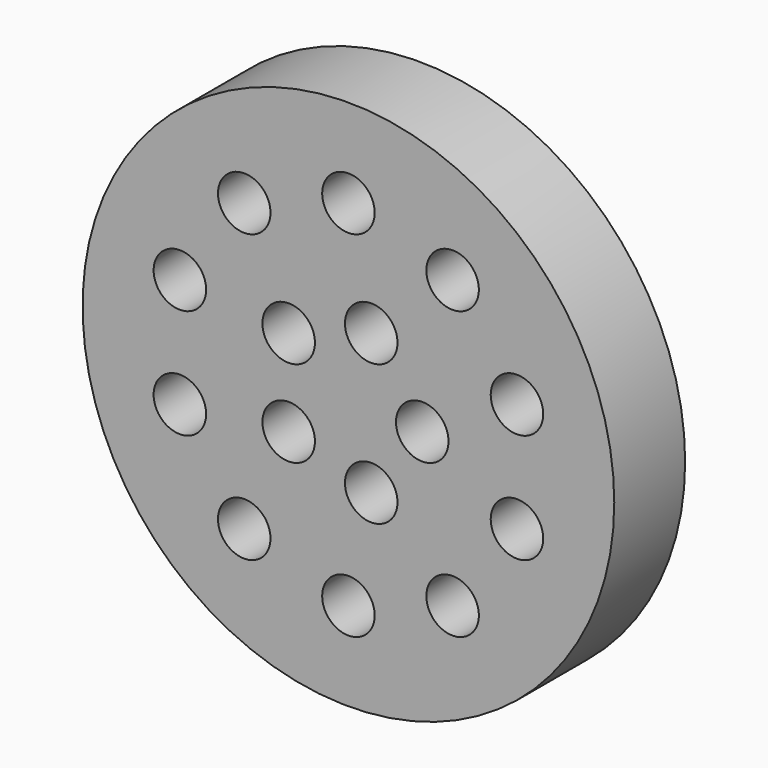
from build123d import *

# Parameters (mm, degrees)
F0_R     = 9
F1_DEPTH = 3
F3_D     = 1.778
F3_DEPTH = 15
F3_TIP   = 0.5341650903


# Not quite as in the source:
# - a feature names something its author has since deleted; it is built from what else it names


with BuildPart() as f1:
    # F0 (on Front) → F1 (new body)
    with BuildSketch(Plane.XZ):
        Circle(F0_R)
    extrude(amount=F1_DEPTH)

    # F3
    with Locations(Plane.XZ.offset(3)):
        with Locations((-3.5267115138, 4.8541019662), (-5.7063390978, 1.8541019662), (-5.7063390978, -1.8541019662), (-3.5267115138, -4.8541019662), (0, -6), (3.5267115138, -4.8541019662), (5.7063390978, -1.8541019662), (0, 6), (-2.0225424859, 1.4694631307), (-2.0225424859, -1.4694631307), (0.7725424859, -2.3776412907), (2.5, 0), (0.7725424859, 2.3776412907), (3.5267115138, 4.8541019662), (5.7063390978, 1.8541019662)):
            Hole(F3_D / 2, depth=F3_DEPTH)
            with Locations((0, 0, -(F3_DEPTH + F3_TIP / 2))):  # 118° drill point
                Cone(0, F3_D / 2, F3_TIP, mode=Mode.SUBTRACT)


solid = f1.part
